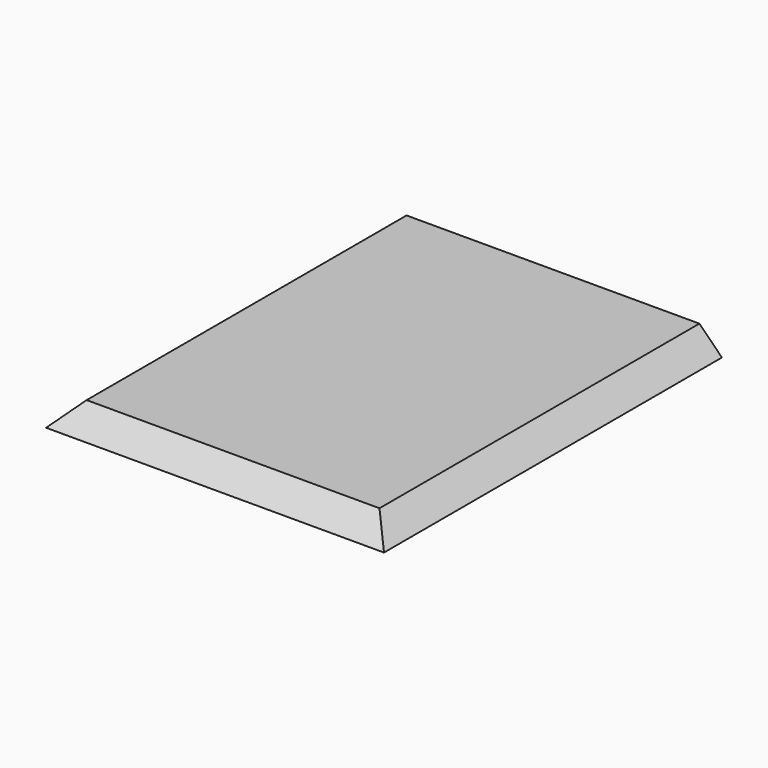
from build123d import *

# Parameters (mm, degrees)
F0_W     = 240
F0_H     = 300
F1_DEPTH = 16
F2_SIZE  = 15.99999


# Not quite as in the source:
# - a fillet or chamfer is up to 0.001 mm smaller than in the source, because OpenCascade refuses the exact size


with BuildPart() as f1:
    # F0 (on Top) → F1 (new body)
    with BuildSketch(Plane.XY):
        with Locations((120, 150)):
            Rectangle(F0_W, F0_H)
    extrude(amount=F1_DEPTH)

    # F2 (size 16 in the source; OpenCascade refuses exactly that, so slightly less here)
    f2_edges = [f1.edges().sort_by_distance(p)[0] for p in [
        (120, 0, 16),
        (240, 150, 16),
        (0, 150, 16),
    ]]
    chamfer(f2_edges, length=F2_SIZE)


solid = f1.part
